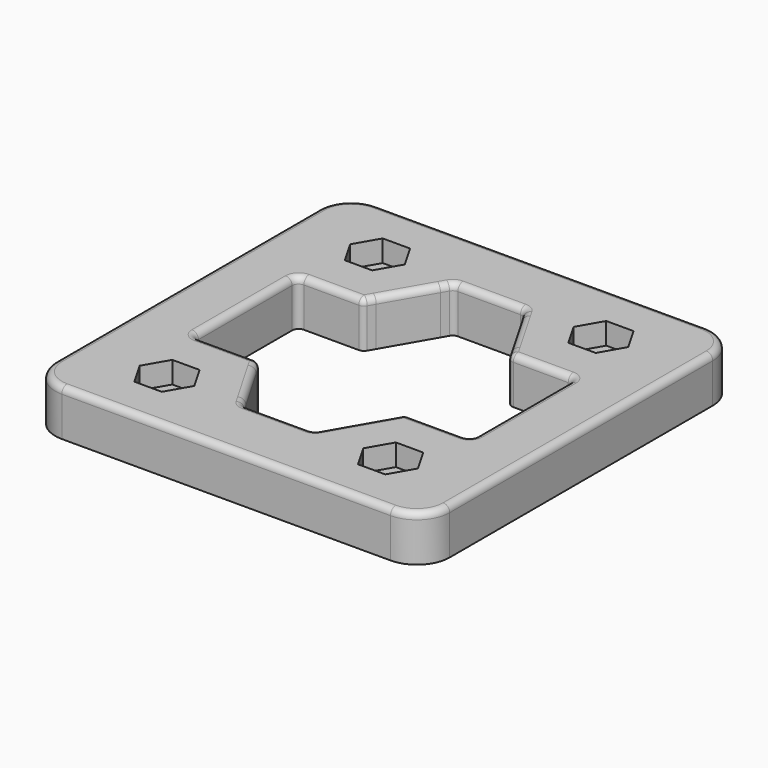
from build123d import *

# Parameters (mm, degrees)
F0_W     = 60
F0_H     = 60
F1_DEPTH = 7
F2_R     = 5
F3_R     = 2.1
F4_DEPTH = 25
F5_DEPTH = 3.3
F6_R     = 1
F7_DEPTH = 25
F8_R     = 1


# Not quite as in the source:
# - a feature names something its author has since deleted; it is built from what else it names


with BuildPart() as f1:
    # F0 (on Top) → F1 (new body)
    with BuildSketch(Plane.XY):
        Rectangle(F0_W, F0_H)
    extrude(amount=-F1_DEPTH)

    # F2
    f2_edges = [f1.edges().sort_by_distance(p)[0] for p in [
        (-30, 30, -3.5),
        (30, 30, -3.5),
        (30, -30, -3.5),
        (-30, -30, -3.5),
    ]]
    fillet(f2_edges, radius=F2_R)

    # F3 (on face) → F4 (cut)
    with BuildSketch(Plane.XY):
        with BuildLine():
            Line((-17, 17.9), (-17, 22.1))
            ThreePointArc((-17, 22.1), (-19.1, 20), (-17, 17.9))
        make_face()
        with BuildLine():
            ThreePointArc((-17, 17.9), (-15.5150757595, 18.5150757595), (-14.9, 20))
            ThreePointArc((-14.9, 20), (-15.5150757595, 21.4849242405), (-17, 22.1))
            Line((-17, 22.1), (-17, 17.9))
        make_face()
        with Locations((17, 20)):
            Circle(F3_R)
        with Locations((17, -20)):
            Circle(F3_R)
        with BuildLine():
            Line((-17, -22.1), (-17, -17.9))
            ThreePointArc((-17, -17.9), (-19.1, -20), (-17, -22.1))
        make_face()
        with BuildLine():
            ThreePointArc((-17, -22.1), (-15.5150757595, -21.4849242405), (-14.9, -20))
            ThreePointArc((-14.9, -20), (-15.5150757595, -18.5150757595), (-17, -17.9))
            Line((-17, -17.9), (-17, -22.1))
        make_face()
    extrude(amount=-F4_DEPTH, mode=Mode.SUBTRACT)

    # F3 (on face) → F5 (cut)
    with BuildSketch(Plane.XY):
        with BuildLine():
            ThreePointArc((-17, 17.9), (-19.1, 20), (-17, 22.1))
            Line((-17, 22.1), (-17, 23.6))
            Line((-17, 23.6), (-19.0784609691, 23.6))
            Line((-19.0784609691, 23.6), (-21.1569219382, 20))
            Line((-21.1569219382, 20), (-19.0784609691, 16.4))
            Line((-19.0784609691, 16.4), (-17, 16.4))
            Line((-17, 16.4), (-17, 17.9))
        make_face()
        with BuildLine():
            ThreePointArc((-17, 22.1), (-15.5150757595, 21.4849242405), (-14.9, 20))
            ThreePointArc((-14.9, 20), (-15.5150757595, 18.5150757595), (-17, 17.9))
            Line((-17, 17.9), (-17, 16.4))
            Line((-17, 16.4), (-14.9215390309, 16.4))
            Line((-14.9215390309, 16.4), (-12.8430780618, 20))
            Line((-12.8430780618, 20), (-14.9215390309, 23.6))
            Line((-14.9215390309, 23.6), (-17, 23.6))
            Line((-17, 23.6), (-17, 22.1))
        make_face()
        Polygon((19.0784609691, 23.6), (14.9215390309, 23.6), (12.8430780618, 20), (14.9215390309, 16.4), (19.0784609691, 16.4), (21.1569219382, 20), align=None)
        with Locations((17, 20)):
            Circle(F3_R, mode=Mode.SUBTRACT)
        with BuildLine():
            ThreePointArc((-17, -22.1), (-19.1, -20), (-17, -17.9))
            Line((-17, -17.9), (-17, -16.4))
            Line((-17, -16.4), (-19.0784609691, -16.4))
            Line((-19.0784609691, -16.4), (-21.1569219382, -20))
            Line((-21.1569219382, -20), (-19.0784609691, -23.6))
            Line((-19.0784609691, -23.6), (-17, -23.6))
            Line((-17, -23.6), (-17, -22.1))
        make_face()
        with BuildLine():
            ThreePointArc((-17, -17.9), (-15.5150757595, -18.5150757595), (-14.9, -20))
            ThreePointArc((-14.9, -20), (-15.5150757595, -21.4849242405), (-17, -22.1))
            Line((-17, -22.1), (-17, -23.6))
            Line((-17, -23.6), (-14.9215390309, -23.6))
            Line((-14.9215390309, -23.6), (-12.8430780618, -20))
            Line((-12.8430780618, -20), (-14.9215390309, -16.4))
            Line((-14.9215390309, -16.4), (-17, -16.4))
            Line((-17, -16.4), (-17, -17.9))
        make_face()
        Polygon((19.0784609691, -23.6), (21.1569219382, -20), (19.0784609691, -16.4), (14.9215390309, -16.4), (12.8430780618, -20), (14.9215390309, -23.6), align=None)
        with Locations((17, -20)):
            Circle(F3_R, mode=Mode.SUBTRACT)
    extrude(amount=-F5_DEPTH, mode=Mode.SUBTRACT)

    # F6
    f6_edges = [f1.edges().sort_by_distance(p)[0] for p in [
        (30, 0, 0),
        (0, 30, 0),
        (-30, 0, 0),
        (0, -30, 0),
        (-28.535534, -28.535534, 0),
        (28.535534, -28.535534, 0),
        (28.535534, 28.535534, 0),
        (-28.535534, 28.535534, 0),
    ]]
    fillet(f6_edges, radius=F6_R)

    # F3 (on face) → F7 (cut)
    with BuildSketch(Plane.XY):
        Polygon((-5.3375245624, 20), (-6.2035499662, 18.5), (-10.3027368774, 11.4), (-11.1687622812, 9.9), (-12.9008130888, 9.9), (-21.0991869112, 9.9), (-21.0991869112, -9.9), (-12.9008130888, -9.9), (-11.1687622812, -9.9), (-10.3027368774, -11.4), (-6.2035499662, -18.5), (-5.3375245624, -20), (5.3375245624, -20), (6.2035499662, -18.5), (10.3027368774, -11.4), (11.1687622812, -9.9), (12.9008130888, -9.9), (21.0991869112, -9.9), (21.0991869112, 9.9), (12.9008130888, 9.9), (11.1687622812, 9.9), (10.3027368774, 11.4), (6.2035499662, 18.5), (5.3375245624, 20), (0, 20), align=None)
    extrude(amount=-F7_DEPTH, mode=Mode.SUBTRACT)

    # F8
    f8_edges = [f1.edges().sort_by_distance(p)[0] for p in [
        (-16.133975, 9.9, 0),
        (-21.099187, 0, 0),
        (-8.253143, 14.95, 0),
        (0, 20, 0),
        (8.253143, 14.95, 0),
        (16.133975, 9.9, 0),
        (21.099187, 0, 0),
        (16.133975, -9.9, 0),
        (8.253143, -14.95, 0),
        (0, -20, 0),
        (-8.253143, -14.95, 0),
        (-16.133975, -9.9, 0),
        (-11.168762, 9.9, -3.5),
        (-5.337525, 20, -3.5),
        (5.337525, 20, -3.5),
        (11.168762, 9.9, -3.5),
        (21.099187, 9.9, -3.5),
        (21.099187, -9.9, -3.5),
        (11.168762, -9.9, -3.5),
        (5.337525, -20, -3.5),
        (-5.337525, -20, -3.5),
        (-11.168762, -9.9, -3.5),
        (-21.099187, -9.9, -3.5),
        (-21.099187, 9.9, -3.5),
    ]]
    fillet(f8_edges, radius=F8_R)


solid = f1.part
